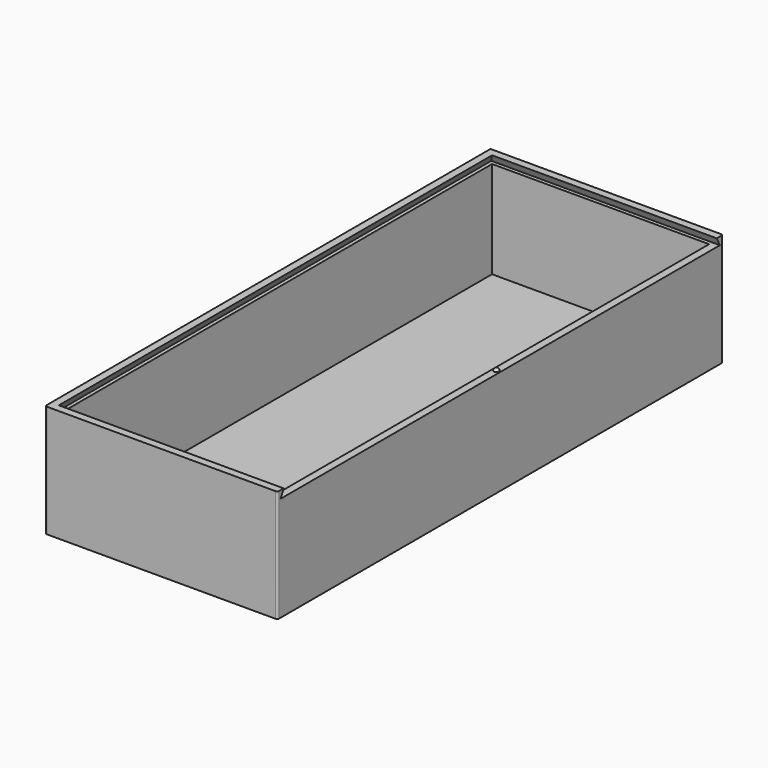
from build123d import *

# Parameters (mm, degrees)
F4_W      = 91
F4_H      = 218
F5_DEPTH  = 41
F8_DEPTH  = 218
F9_DEPTH  = 91
F10_W     = 85
F10_H     = 212
F11_DEPTH = 38
F12_R     = 0.75


with BuildPart() as f5:
    # F4 (on Top) → F5 (new body)
    with BuildSketch(Plane.XY):
        with Locations((45.5, 109)):
            Rectangle(F4_W, F4_H)
    extrude(amount=F5_DEPTH)

    # F7 (on face) → F8 (join)
    with BuildSketch(Plane.XZ):
        Polygon((0, 44), (0, 41), (1.5, 41), (3, 44), align=None)
    extrude(amount=-F8_DEPTH)

    # F6 (on face) → F9 (join)
    with BuildSketch(Plane.YZ.offset(91)):
        Polygon((0, 44), (0, 41), (1.5, 41), (3, 44), align=None)
        Polygon((216.5, 41), (218, 41), (218, 44), (215, 44), align=None)
    extrude(amount=-F9_DEPTH)

    # F10 (on face) → F11 (cut)
    with BuildSketch(Plane.XY.offset(41)):
        with Locations((45.5, 109)):
            Rectangle(F10_W, F10_H)
    extrude(amount=-F11_DEPTH, mode=Mode.SUBTRACT)

    # F12
    f12_edges = [f5.edges().sort_by_distance(p)[0] for p in [
        (91, 0, 22),
        (91, 218, 22),
        (0, 0, 22),
    ]]
    fillet(f12_edges, radius=F12_R)

    # F13 (on face) → F14 (revolve)
    with BuildSketch(Plane.XY.offset(41)):
        with BuildLine():
            Line((88.5, 109), (90.5, 109))
            ThreePointArc((90.5, 109), (89.5, 110), (88.5, 109))
        make_face()
    revolve(axis=Axis((24.0288835471, 109, 41), (-1, 0, 0)))


solid = f5.part
